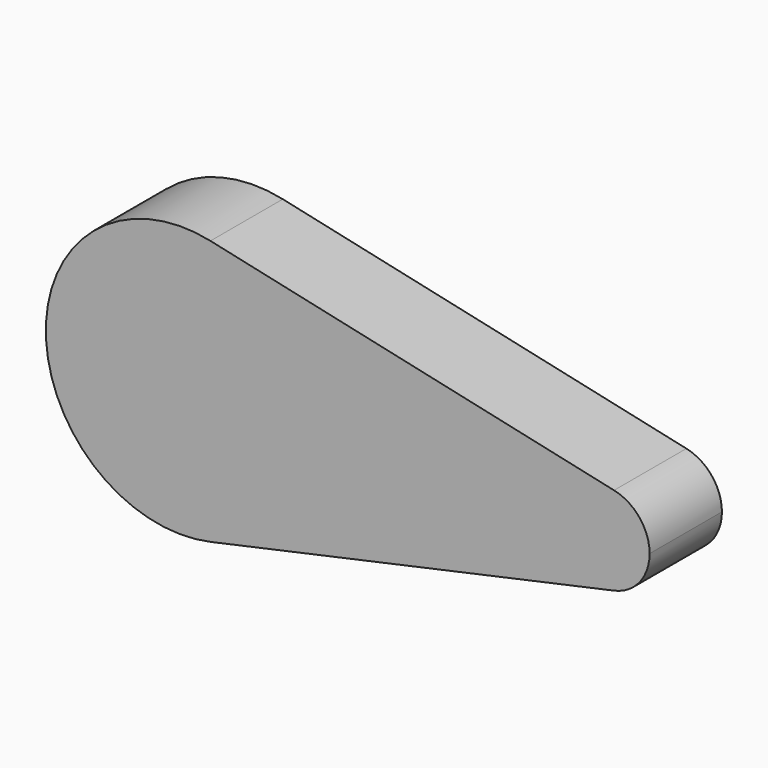
from build123d import *

# Parameters (mm, degrees)
F1_DEPTH = 25.4


# Not quite as in the source:
# - the program builds the solid bodies; features that only make, move or delete a surface that nothing else refers to are left out


with BuildPart() as f1:
    # F0 (on Front) → F1 (new body)
    with BuildSketch(Plane.XZ):
        with BuildLine():
            ThreePointArc((8.1449308648, -37.2192168269), (29.6810702801, -23.888157464), (38.1, 0))
            ThreePointArc((38.1, 0), (29.6810702801, 23.888157464), (8.1449308648, 37.2192168269))
            ThreePointArc((8.1449308648, 37.2192168269), (-38.1, 0), (8.1449308648, -37.2192168269))
        make_face()
        with BuildLine():
            ThreePointArc((131.5150048256, 0), (128.708694919, 7.9627191547), (121.5299817805, 12.406405609))
            ThreePointArc((121.5299817805, 12.406405609), (106.1150048256, 0), (121.5299817805, -12.406405609))
            ThreePointArc((121.5299817805, -12.406405609), (128.708694919, -7.9627191547), (131.5150048256, 0))
        make_face()
        with BuildLine():
            ThreePointArc((8.1449308648, 37.2192168269), (29.6810702801, 23.888157464), (38.1, 0))
            ThreePointArc((38.1, 0), (29.6810702801, -23.888157464), (8.1449308648, -37.2192168269))
            Line((8.1449308648, -37.2192168269), (121.5299817805, -12.406405609))
            ThreePointArc((121.5299817805, -12.406405609), (106.1150048256, 0), (121.5299817805, 12.406405609))
            Line((121.5299817805, 12.406405609), (8.1449308648, 37.2192168269))
        make_face()
    extrude(amount=F1_DEPTH)


solid = f1.part
